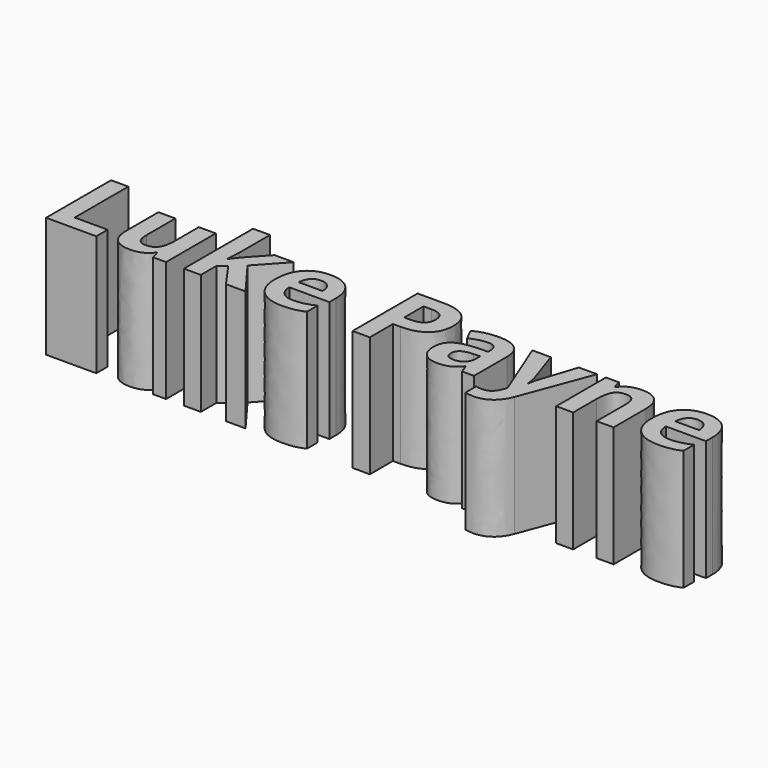
from build123d import *

# Parameters (mm, degrees)
F0_TEXT_SIZE = 93.426855488
F1_DEPTH     = 99


# Not quite as in the source:
# - Text() gives the source's letters only with a copy of the font that has no kerning and outlines rounded to 1/6400 em; it was checked with that copy


with BuildPart() as f1:
    # F0 (on Top) → F1 (new body)
    with BuildSketch(Plane.XY):
        with Locations((26.5375133604, 0)):
            Text('Luke Payne', F0_TEXT_SIZE, font='Open Sans', font_style=FontStyle.BOLD, text_align=(TextAlign.LEFT, TextAlign.BOTTOM))
    extrude(amount=-F1_DEPTH)


solid = f1.part
